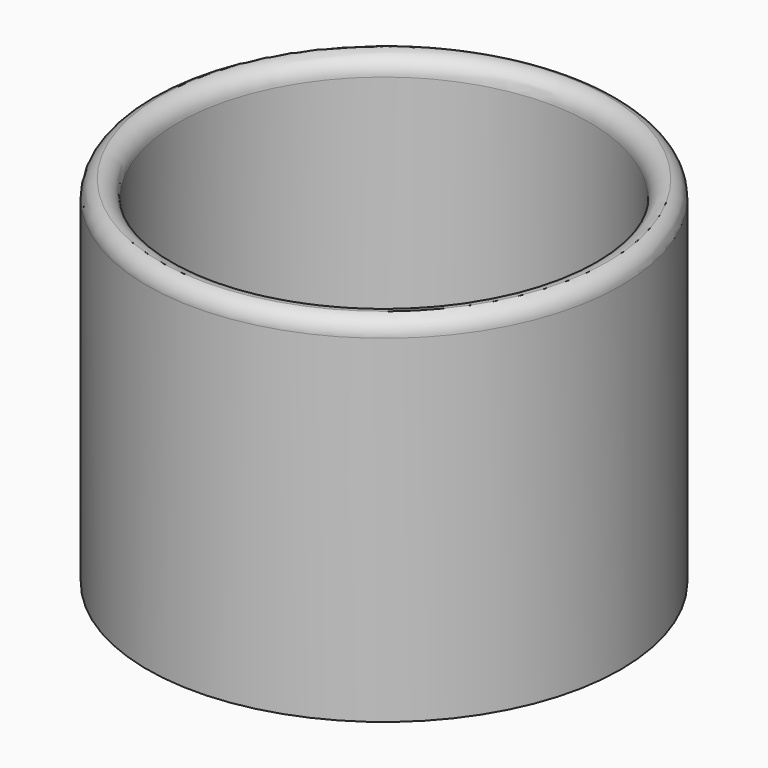
from build123d import *

# Parameters (mm, degrees)
F2_R = 5.08
F3_R = 5.08


# Not quite as in the source:
# - a fillet or chamfer that OpenCascade refuses, or shapes differently, is made with other operations: its cross-section is extruded or revolved along the edge and cut away or added


with BuildPart() as f1:
    # F0 (on Front) → F1 (revolve)
    with BuildSketch(Plane.XZ):
        Polygon((68.2647973299, 48.6955605447), (59.4662241638, 48.6955605447), (59.4662241638, -48.6955568194), (0, -60.2247230709), (0, -68.4164986014), (68.2647973299, -53.5499453545), align=None)
    revolve(axis=Axis((0, 0, 0.9102020413), (0, 0, -1)))

    # F2
    f2_edges = [f1.edges().sort_by_distance(p)[0] for p in [
        (-59.466224, 0, -48.695557),
        (29.733112, 0, -54.46014),
    ]]
    fillet(f2_edges, radius=F2_R)

    # F3
    f3_edges = [f1.edges().sort_by_distance(p)[0] for p in [
        (-59.466224, 0, 48.695561),
    ]]
    fillet(f3_edges, radius=F3_R)

    # F4: fillet of radius 5.08 on 1 edges, made by hand

    # F4_s1 → F4_t2 (revolve, cut)
    with BuildSketch(Plane.XZ):
        with BuildLine():
            ThreePointArc((64.5462241638, 48.6955605447), (67.2296983371, 46.8746892895), (68.2647973299, 43.8013888093))
            Line((68.2647973299, 43.8013888093), (68.2647973299, 48.6955605447))
            Line((68.2647973299, 48.6955605447), (64.5462241638, 48.6955605447))
        make_face()
    revolve(axis=Axis((0, 0, 48.6955605447), (0, 0, -1)), mode=Mode.SUBTRACT)


solid = f1.part
